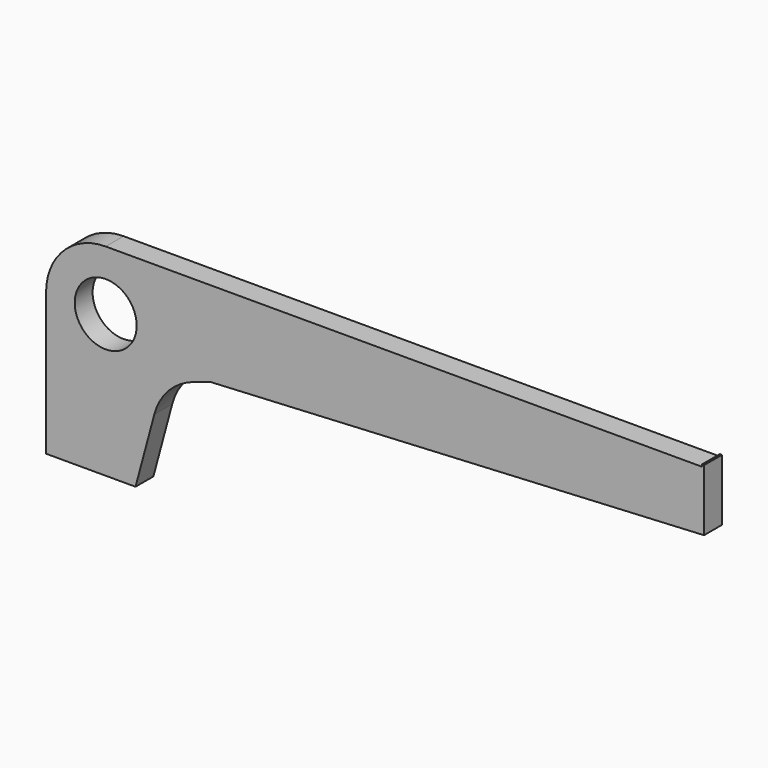
from build123d import *

# Parameters (mm, degrees)
F1_DEPTH = 2.38125
F2_R     = 3.2981725782
F3_DEPTH = 25.4


# Not quite as in the source:
# - a length typed as a fraction of an inch, garbled in the dataset ("3 / 203.2 mm" for 3/8 in), is restored


with BuildPart() as f1:
    # F0 (on Front) → F1 (new body)
    with BuildSketch(Plane.XZ):
        with BuildLine():
            Line((69.85, 21.4939358442), (6.35, 21.4939358442))
            ThreePointArc((6.35, 21.4939358442), (1.8598719395, 19.6340639047), (0, 15.1439358442))
            Line((0, 15.1439358442), (0, 0))
            Line((0, 0), (9.525, 0))
            Line((9.525, 0), (11.5292743985, 7.4402281731))
            ThreePointArc((11.5292743985, 7.4402281731), (13.0480987591, 10.1527436206), (15.6724793239, 11.8192351874))
            Line((15.6724793239, 11.8192351874), (17.4910178831, 12.4187755322))
            Line((17.4910178831, 12.4187755322), (70.0698060278, 15.1439358442))
            Line((70.0698060278, 15.1439358442), (69.85, 15.1439358442))
            Line((69.85, 15.1439358442), (69.85, 21.4939358442))
        make_face()
        Polygon((69.85, 21.7137452919), (69.85, 21.4939358442), (69.85, 15.1439358442), (70.0698060278, 15.1439358442), (70.0698060278, 21.7137452919), align=None)
    extrude(amount=F1_DEPTH)

    # F2 (on face) → F3 (cut)
    with BuildSketch(Plane.XZ.offset(2.38125)):
        with Locations((6.35, 15.1439358442)):
            Circle(F2_R)
    extrude(amount=-F3_DEPTH, mode=Mode.SUBTRACT)


solid = f1.part
